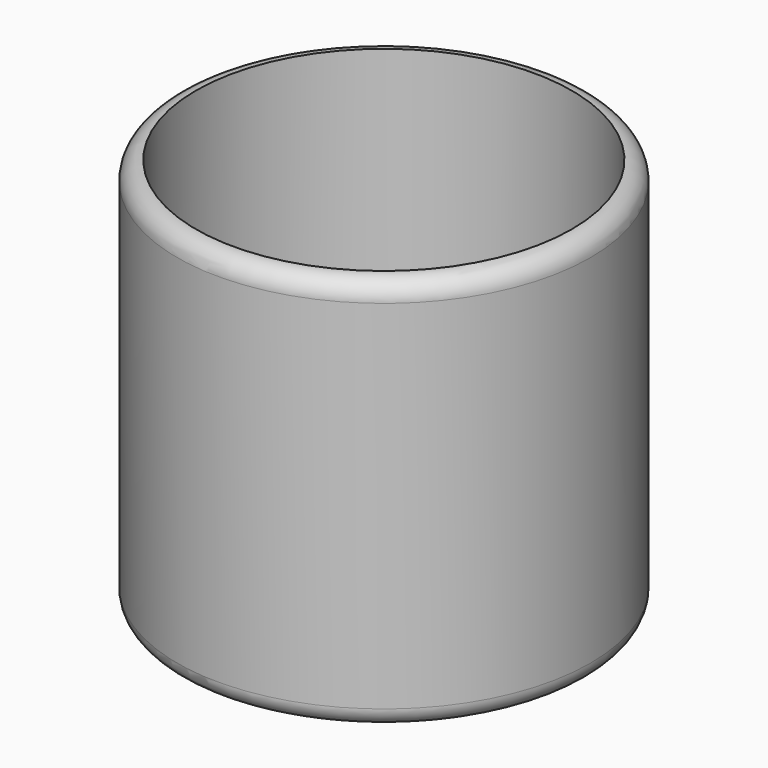
from build123d import *

# Parameters (mm, degrees)
F0_R     = 50
F1_DEPTH = 100
F2_T     = 5


# Not quite as in the source:
# - a fillet or chamfer that OpenCascade refuses, or shapes differently, is made with other operations: its cross-section is extruded or revolved along the edge and cut away or added
# - a feature of the source that left no trace in its solid (it failed there, or was rolled back) is left out


with BuildPart() as f1:
    # F0 (on Top) → F1 (new body)
    with BuildSketch(Plane.XY):
        Circle(F0_R)
    extrude(amount=F1_DEPTH)

    # F2
    f2_openings = [f1.faces().sort_by_distance(p)[0] for p in [
        (0, 0, 100),
    ]]
    offset(amount=F2_T, openings=f2_openings, kind=Kind.INTERSECTION)

    # F3: fillet of radius 5 on 2 edges, made by hand

    # F3_s1 → F3_t2 (revolve, cut)
    with BuildSketch(Plane.XZ):
        with BuildLine():
            ThreePointArc((50, 100), (53.5355339059, 98.5355339059), (55, 95))
            Line((55, 95), (55, 100))
            Line((55, 100), (50, 100))
        make_face()
    revolve(axis=Axis((0, 0, 100), (0, 0, -1)), mode=Mode.SUBTRACT)

    # F3_s3 → F3_t4 (revolve, cut)
    with BuildSketch(Plane.XZ):
        with BuildLine():
            ThreePointArc((55, 0), (53.5355339059, -3.5355339059), (50, -5))
            Line((50, -5), (55, -5))
            Line((55, -5), (55, 0))
        make_face()
    revolve(axis=Axis((0, 0, -5), (0, 0, -1)), mode=Mode.SUBTRACT)


solid = f1.part
